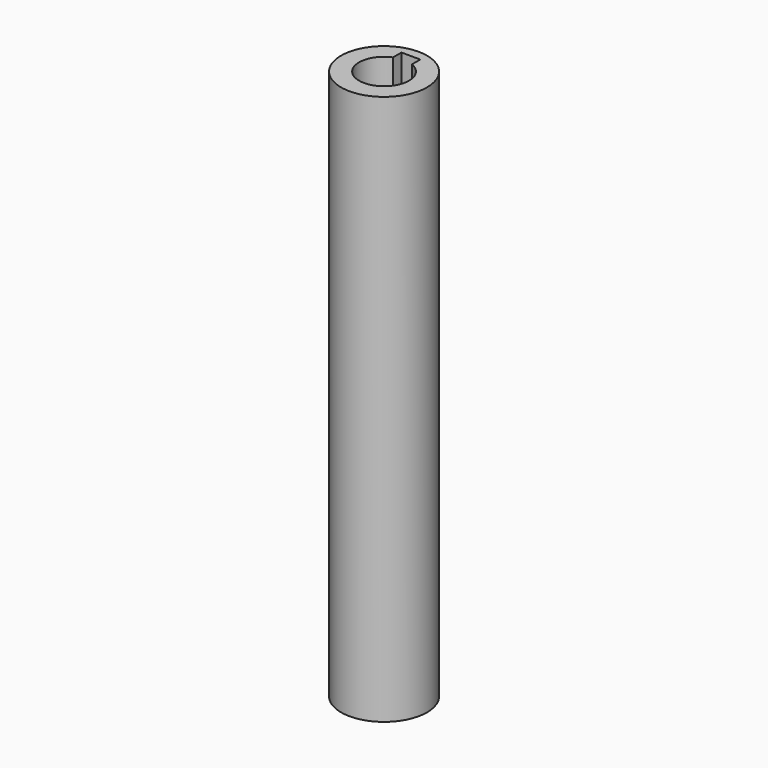
from build123d import *

# Parameters (mm, degrees)
F0_R     = 12.5
F1_DEPTH = 160
F3_DEPTH = 40


# Not quite as in the source:
# - a feature names something its author has since deleted; it is built from what else it names


with BuildPart() as f1:
    # F0 (on Top) → F1 (new body)
    with BuildSketch(Plane.XY):
        Circle(F0_R)
    extrude(amount=F1_DEPTH)

    # F2 (on face) → F3 (cut)
    with BuildSketch(Plane.XY.offset(160)):
        with BuildLine():
            ThreePointArc((-2.75, 6.7082039325), (-4.0388736054, -6.0207972894), (7.25, 0))
            ThreePointArc((7.25, 0), (6.0207972894, 4.0388736054), (2.75, 6.7082039325))
            Line((2.75, 6.7082039325), (2.75, 4.75))
            Line((2.75, 4.75), (-2.75, 4.75))
            Line((-2.75, 4.75), (-2.75, 6.7082039325))
        make_face()
        with BuildLine():
            Line((2.75, 4.75), (2.75, 6.7082039325))
            ThreePointArc((2.75, 6.7082039325), (0, 7.25), (-2.75, 6.7082039325))
            Line((-2.75, 6.7082039325), (-2.75, 4.75))
            Line((-2.75, 4.75), (2.75, 4.75))
        make_face()
        with BuildLine():
            ThreePointArc((-2.75, 6.7082039325), (0, 7.25), (2.75, 6.7082039325))
            Line((2.75, 6.7082039325), (2.75, 9.75))
            Line((2.75, 9.75), (-2.75, 9.75))
            Line((-2.75, 9.75), (-2.75, 6.7082039325))
        make_face()
    extrude(amount=-F3_DEPTH, mode=Mode.SUBTRACT)


solid = f1.part
